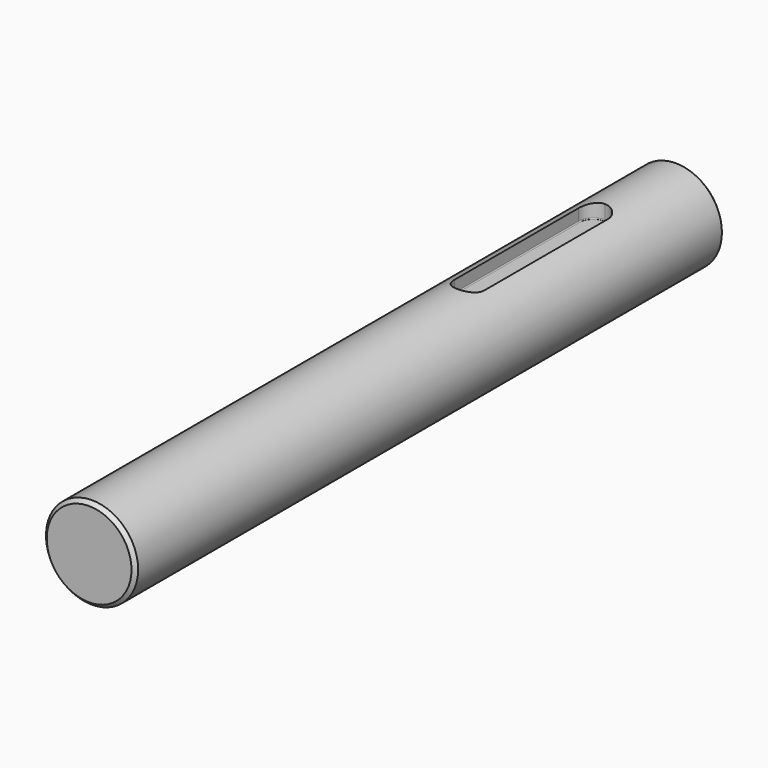
from build123d import *

# Parameters (mm, degrees)
F0_R     = 12.5
F1_DEPTH = 200
F3_W     = 8
F3_H     = 50
F4_DEPTH = 4
F5_R     = 3.9999
F6_R     = 0.25
F7_SIZE  = 1


# Not quite as in the source:
# - a fillet or chamfer is up to 0.001 mm smaller than in the source, because OpenCascade refuses the exact size


with BuildPart() as f1:
    # F0 (on Front) → F1 (new body)
    with BuildSketch(Plane.XZ):
        Circle(F0_R)
    extrude(amount=F1_DEPTH)

    # F3 (on offset) → F4 (cut)
    with BuildSketch(Plane.XY.offset(12.5)):
        with Locations((0, -50)):
            Rectangle(F3_W, F3_H)
    extrude(amount=-F4_DEPTH, mode=Mode.SUBTRACT)

    # F5 (radius 4 in the source; OpenCascade refuses exactly that, so slightly less here)
    f5_edges = [f1.edges().sort_by_distance(p)[0] for p in [
        (-4, -25, 10.17136),
        (4, -25, 10.17136),
        (4, -75, 10.17136),
        (-4, -75, 10.17136),
    ]]
    fillet(f5_edges, radius=F5_R)

    # F6
    f6_edges = [f1.edges().sort_by_distance(p)[0] for p in [
        (0, -25, 8.5),
        (2.828456, -26.171544, 8.5),
        (-2.828456, -26.171544, 8.5),
        (4, -50, 8.5),
        (-4, -50, 8.5),
        (2.828456, -73.828456, 8.5),
        (-2.828456, -73.828456, 8.5),
        (0, -75, 8.5),
    ]]
    fillet(f6_edges, radius=F6_R)

    # F7
    f7_edges = [f1.edges().sort_by_distance(p)[0] for p in [
        (-12.5, -200, 0),
        (-12.5, 0, 0),
    ]]
    chamfer(f7_edges, length=F7_SIZE)


solid = f1.part
